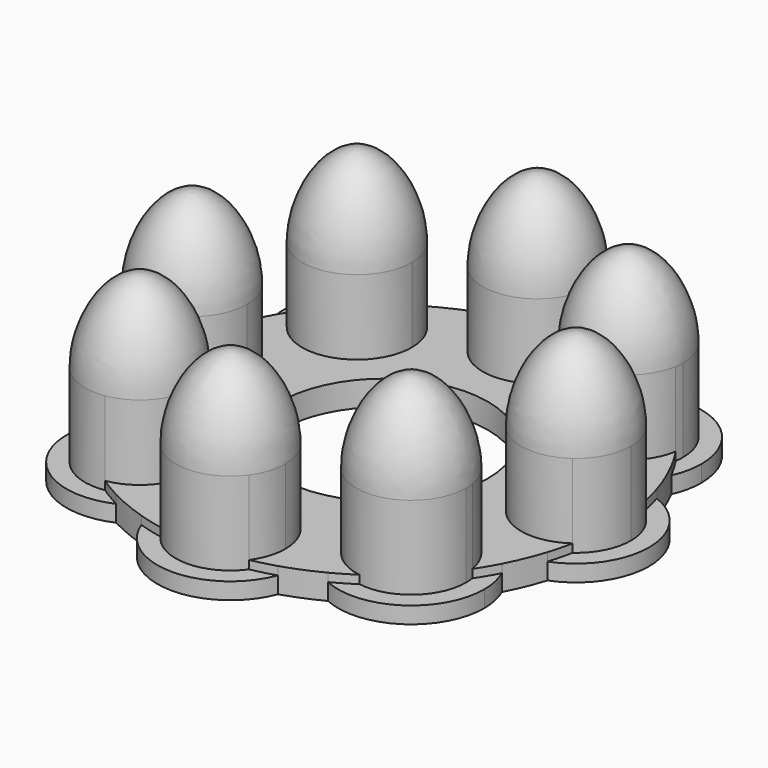
from build123d import *

# Parameters (mm, degrees)
F0_R            = 7.9375
F1_DEPTH        = 0.635
F2_DEPTH        = 1.27
F3_DEPTH        = 6.35
F5_COPIES_COUNT = 8


# Not quite as in the source:
# - a pattern or mirror of a feature is missing from the dataset's text; its kind, count and spacing are read off the source's solid


with BuildPart() as f1:
    # F0 (on Top) → F1 (new body)
    with BuildSketch(Plane.XY):
        with BuildLine():
            ThreePointArc((-5.219470135, 16.6642142857), (-1.0147277679, 9.1734047727), (5.588, 14.6685))
            ThreePointArc((5.588, 14.6685), (5.4950952273, 15.6832277679), (5.219470135, 16.6642142857))
            ThreePointArc((5.219470135, 16.6642142857), (4.3120566918, 16.9217337568), (3.3920620288, 17.1298809524))
            ThreePointArc((3.3920620288, 17.1298809524), (3.986264728, 15.96239896), (4.191, 14.6685))
            ThreePointArc((4.191, 14.6685), (-1.29389896, 10.682235272), (-3.3920620288, 17.1298809524))
            ThreePointArc((-3.3920620288, 17.1298809524), (-4.3120566918, 16.9217337568), (-5.219470135, 16.6642142857))
        make_face()
        with BuildLine():
            ThreePointArc((9.7141049196, 14.5112050451), (8.9163881613, 15.0145572165), (8.0926561979, 15.4741016512))
            ThreePointArc((8.0926561979, 15.4741016512), (6.4208831266, 6.4208831266), (15.4741016512, 8.0926561979))
            ThreePointArc((15.4741016512, 8.0926561979), (15.0145572165, 8.9163881613), (14.5112050451, 9.7141049196))
            ThreePointArc((14.5112050451, 9.7141049196), (7.4087112999, 7.4087112999), (9.7141049196, 14.5112050451))
        make_face()
        with BuildLine():
            ThreePointArc((17.1298809524, 3.3920620288), (16.9217337568, 4.3120566918), (16.6642142857, 5.219470135))
            ThreePointArc((16.6642142857, 5.219470135), (9.0805, 0), (16.6642142857, -5.219470135))
            ThreePointArc((16.6642142857, -5.219470135), (16.9217337568, -4.3120566918), (17.1298809524, -3.3920620288))
            ThreePointArc((17.1298809524, -3.3920620288), (10.4775, 0), (17.1298809524, 3.3920620288))
        make_face()
        with BuildLine():
            ThreePointArc((14.5112050451, -9.7141049196), (15.0145572165, -8.9163881613), (15.4741016512, -8.0926561979))
            ThreePointArc((15.4741016512, -8.0926561979), (6.4208831266, -6.4208831266), (8.0926561979, -15.4741016512))
            ThreePointArc((8.0926561979, -15.4741016512), (8.9163881613, -15.0145572165), (9.7141049196, -14.5112050451))
            ThreePointArc((9.7141049196, -14.5112050451), (7.4087112999, -7.4087112999), (14.5112050451, -9.7141049196))
        make_face()
        with BuildLine():
            ThreePointArc((3.3920620288, -17.1298809524), (4.3120566918, -16.9217337568), (5.219470135, -16.6642142857))
            ThreePointArc((5.219470135, -16.6642142857), (5.4950952273, -15.6832277679), (5.588, -14.6685))
            ThreePointArc((5.588, -14.6685), (-1.0147277679, -9.1734047727), (-5.219470135, -16.6642142857))
            ThreePointArc((-5.219470135, -16.6642142857), (-4.3120566918, -16.9217337568), (-3.3920620288, -17.1298809524))
            ThreePointArc((-3.3920620288, -17.1298809524), (-1.29389896, -10.682235272), (4.191, -14.6685))
            ThreePointArc((4.191, -14.6685), (3.986264728, -15.96239896), (3.3920620288, -17.1298809524))
        make_face()
        with BuildLine():
            ThreePointArc((-4.7841958198, -10.3721958198), (-9.2068001329, -4.907070305), (-15.4741016512, -8.0926561979))
            ThreePointArc((-15.4741016512, -8.0926561979), (-15.0145572165, -8.9163881613), (-14.5112050451, -9.7141049196))
            ThreePointArc((-14.5112050451, -9.7141049196), (-10.0421251177, -6.1942137314), (-6.1811958198, -10.3721958198))
            ThreePointArc((-6.1811958198, -10.3721958198), (-7.1845211216, -13.0930800545), (-9.7141049196, -14.5112050451))
            ThreePointArc((-9.7141049196, -14.5112050451), (-8.9163881613, -15.0145572165), (-8.0926561979, -15.4741016512))
            ThreePointArc((-8.0926561979, -15.4741016512), (-5.6837093153, -13.4125639384), (-4.7841958198, -10.3721958198))
        make_face()
        with BuildLine():
            ThreePointArc((-9.0805, 0), (-11.5004017872, 4.6031399842), (-16.6642142857, 5.219470135))
            ThreePointArc((-16.6642142857, 5.219470135), (-16.9217337568, 4.3120566918), (-17.1298809524, 3.3920620288))
            ThreePointArc((-17.1298809524, 3.3920620288), (-12.764709908, 3.7336395495), (-10.4775, 0))
            ThreePointArc((-10.4775, 0), (-12.764709908, -3.7336395495), (-17.1298809524, -3.3920620288))
            ThreePointArc((-17.1298809524, -3.3920620288), (-16.9217337568, -4.3120566918), (-16.6642142857, -5.219470135))
            ThreePointArc((-16.6642142857, -5.219470135), (-11.5004017872, -4.6031399842), (-9.0805, 0))
        make_face()
        with BuildLine():
            ThreePointArc((-4.7841958198, 10.3721958198), (-5.6837093153, 13.4125639384), (-8.0926561979, 15.4741016512))
            ThreePointArc((-8.0926561979, 15.4741016512), (-8.9163881613, 15.0145572165), (-9.7141049196, 14.5112050451))
            ThreePointArc((-9.7141049196, 14.5112050451), (-7.1845211216, 13.0930800545), (-6.1811958198, 10.3721958198))
            ThreePointArc((-6.1811958198, 10.3721958198), (-10.0421251177, 6.1942137314), (-14.5112050451, 9.7141049196))
            ThreePointArc((-14.5112050451, 9.7141049196), (-15.0145572165, 8.9163881613), (-15.4741016512, 8.0926561979))
            ThreePointArc((-15.4741016512, 8.0926561979), (-9.2068001329, 4.907070305), (-4.7841958198, 10.3721958198))
        make_face()
        with BuildLine():
            ThreePointArc((5.219470135, 16.6642142857), (5.4950952273, 15.6832277679), (5.588, 14.6685))
            ThreePointArc((5.588, 14.6685), (-1.0147277679, 9.1734047727), (-5.219470135, 16.6642142857))
            ThreePointArc((-5.219470135, 16.6642142857), (-6.6826094377, 16.1332463365), (-8.0926561979, 15.4741016512))
            ThreePointArc((-8.0926561979, 15.4741016512), (-5.6837093153, 13.4125639384), (-4.7841958198, 10.3721958198))
            ThreePointArc((-4.7841958198, 10.3721958198), (-9.2068001329, 4.907070305), (-15.4741016512, 8.0926561979))
            ThreePointArc((-15.4741016512, 8.0926561979), (-16.1332463365, 6.6826094377), (-16.6642142857, 5.219470135))
            ThreePointArc((-16.6642142857, 5.219470135), (-11.5004017872, 4.6031399842), (-9.0805, 0))
            ThreePointArc((-9.0805, 0), (-11.5004017872, -4.6031399842), (-16.6642142857, -5.219470135))
            ThreePointArc((-16.6642142857, -5.219470135), (-16.1332463365, -6.6826094377), (-15.4741016512, -8.0926561979))
            ThreePointArc((-15.4741016512, -8.0926561979), (-9.2068001329, -4.907070305), (-4.7841958198, -10.3721958198))
            ThreePointArc((-4.7841958198, -10.3721958198), (-5.6837093153, -13.4125639384), (-8.0926561979, -15.4741016512))
            ThreePointArc((-8.0926561979, -15.4741016512), (-6.6826094377, -16.1332463365), (-5.219470135, -16.6642142857))
            ThreePointArc((-5.219470135, -16.6642142857), (-1.0147277679, -9.1734047727), (5.588, -14.6685))
            ThreePointArc((5.588, -14.6685), (5.4950952273, -15.6832277679), (5.219470135, -16.6642142857))
            ThreePointArc((5.219470135, -16.6642142857), (6.6826094377, -16.1332463365), (8.0926561979, -15.4741016512))
            ThreePointArc((8.0926561979, -15.4741016512), (6.4208831266, -6.4208831266), (15.4741016512, -8.0926561979))
            ThreePointArc((15.4741016512, -8.0926561979), (16.1332463365, -6.6826094377), (16.6642142857, -5.219470135))
            ThreePointArc((16.6642142857, -5.219470135), (9.0805, 0), (16.6642142857, 5.219470135))
            ThreePointArc((16.6642142857, 5.219470135), (16.1332463365, 6.6826094377), (15.4741016512, 8.0926561979))
            ThreePointArc((15.4741016512, 8.0926561979), (6.4208831266, 6.4208831266), (8.0926561979, 15.4741016512))
            ThreePointArc((8.0926561979, 15.4741016512), (6.6826094377, 16.1332463365), (5.219470135, 16.6642142857))
        make_face()
        Circle(F0_R, mode=Mode.SUBTRACT)
    extrude(amount=F1_DEPTH)

    # F0 (on Top) → F2 (join)
    with BuildSketch(Plane.XY):
        with BuildLine():
            ThreePointArc((-5.219470135, 16.6642142857), (-1.0147277679, 9.1734047727), (5.588, 14.6685))
            ThreePointArc((5.588, 14.6685), (5.4950952273, 15.6832277679), (5.219470135, 16.6642142857))
            ThreePointArc((5.219470135, 16.6642142857), (4.3120566918, 16.9217337568), (3.3920620288, 17.1298809524))
            ThreePointArc((3.3920620288, 17.1298809524), (3.986264728, 15.96239896), (4.191, 14.6685))
            ThreePointArc((4.191, 14.6685), (-1.29389896, 10.682235272), (-3.3920620288, 17.1298809524))
            ThreePointArc((-3.3920620288, 17.1298809524), (-4.3120566918, 16.9217337568), (-5.219470135, 16.6642142857))
        make_face()
        with BuildLine():
            ThreePointArc((5.219470135, 16.6642142857), (5.4950952273, 15.6832277679), (5.588, 14.6685))
            ThreePointArc((5.588, 14.6685), (-1.0147277679, 9.1734047727), (-5.219470135, 16.6642142857))
            ThreePointArc((-5.219470135, 16.6642142857), (-6.6826094377, 16.1332463365), (-8.0926561979, 15.4741016512))
            ThreePointArc((-8.0926561979, 15.4741016512), (-5.6837093153, 13.4125639384), (-4.7841958198, 10.3721958198))
            ThreePointArc((-4.7841958198, 10.3721958198), (-9.2068001329, 4.907070305), (-15.4741016512, 8.0926561979))
            ThreePointArc((-15.4741016512, 8.0926561979), (-16.1332463365, 6.6826094377), (-16.6642142857, 5.219470135))
            ThreePointArc((-16.6642142857, 5.219470135), (-11.5004017872, 4.6031399842), (-9.0805, 0))
            ThreePointArc((-9.0805, 0), (-11.5004017872, -4.6031399842), (-16.6642142857, -5.219470135))
            ThreePointArc((-16.6642142857, -5.219470135), (-16.1332463365, -6.6826094377), (-15.4741016512, -8.0926561979))
            ThreePointArc((-15.4741016512, -8.0926561979), (-9.2068001329, -4.907070305), (-4.7841958198, -10.3721958198))
            ThreePointArc((-4.7841958198, -10.3721958198), (-5.6837093153, -13.4125639384), (-8.0926561979, -15.4741016512))
            ThreePointArc((-8.0926561979, -15.4741016512), (-6.6826094377, -16.1332463365), (-5.219470135, -16.6642142857))
            ThreePointArc((-5.219470135, -16.6642142857), (-1.0147277679, -9.1734047727), (5.588, -14.6685))
            ThreePointArc((5.588, -14.6685), (5.4950952273, -15.6832277679), (5.219470135, -16.6642142857))
            ThreePointArc((5.219470135, -16.6642142857), (6.6826094377, -16.1332463365), (8.0926561979, -15.4741016512))
            ThreePointArc((8.0926561979, -15.4741016512), (6.4208831266, -6.4208831266), (15.4741016512, -8.0926561979))
            ThreePointArc((15.4741016512, -8.0926561979), (16.1332463365, -6.6826094377), (16.6642142857, -5.219470135))
            ThreePointArc((16.6642142857, -5.219470135), (9.0805, 0), (16.6642142857, 5.219470135))
            ThreePointArc((16.6642142857, 5.219470135), (16.1332463365, 6.6826094377), (15.4741016512, 8.0926561979))
            ThreePointArc((15.4741016512, 8.0926561979), (6.4208831266, 6.4208831266), (8.0926561979, 15.4741016512))
            ThreePointArc((8.0926561979, 15.4741016512), (6.6826094377, 16.1332463365), (5.219470135, 16.6642142857))
        make_face()
        Circle(F0_R, mode=Mode.SUBTRACT)
        with BuildLine():
            ThreePointArc((3.3920620288, 17.1298809524), (4.3120566918, 16.9217337568), (5.219470135, 16.6642142857))
            ThreePointArc((5.219470135, 16.6642142857), (0, 20.2565), (-5.219470135, 16.6642142857))
            ThreePointArc((-5.219470135, 16.6642142857), (-4.3120566918, 16.9217337568), (-3.3920620288, 17.1298809524))
            ThreePointArc((-3.3920620288, 17.1298809524), (0, 18.8595), (3.3920620288, 17.1298809524))
        make_face()
        with BuildLine():
            ThreePointArc((15.9601958198, 10.3721958198), (13.4125639384, 15.0606823244), (8.0926561979, 15.4741016512))
            ThreePointArc((8.0926561979, 15.4741016512), (8.9163881613, 15.0145572165), (9.7141049196, 14.5112050451))
            ThreePointArc((9.7141049196, 14.5112050451), (13.0930800545, 13.559870518), (14.5631958198, 10.3721958198))
            ThreePointArc((14.5631958198, 10.3721958198), (14.5501779083, 10.0421251177), (14.5112050451, 9.7141049196))
            ThreePointArc((14.5112050451, 9.7141049196), (15.0145572165, 8.9163881613), (15.4741016512, 8.0926561979))
            ThreePointArc((15.4741016512, 8.0926561979), (15.8373213347, 9.2068001329), (15.9601958198, 10.3721958198))
        make_face()
        with BuildLine():
            ThreePointArc((9.7141049196, 14.5112050451), (8.9163881613, 15.0145572165), (8.0926561979, 15.4741016512))
            ThreePointArc((8.0926561979, 15.4741016512), (6.4208831266, 6.4208831266), (15.4741016512, 8.0926561979))
            ThreePointArc((15.4741016512, 8.0926561979), (15.0145572165, 8.9163881613), (14.5112050451, 9.7141049196))
            ThreePointArc((14.5112050451, 9.7141049196), (7.4087112999, 7.4087112999), (9.7141049196, 14.5112050451))
        make_face()
        with BuildLine():
            ThreePointArc((-4.7841958198, 10.3721958198), (-5.6837093153, 13.4125639384), (-8.0926561979, 15.4741016512))
            ThreePointArc((-8.0926561979, 15.4741016512), (-8.9163881613, 15.0145572165), (-9.7141049196, 14.5112050451))
            ThreePointArc((-9.7141049196, 14.5112050451), (-7.1845211216, 13.0930800545), (-6.1811958198, 10.3721958198))
            ThreePointArc((-6.1811958198, 10.3721958198), (-10.0421251177, 6.1942137314), (-14.5112050451, 9.7141049196))
            ThreePointArc((-14.5112050451, 9.7141049196), (-15.0145572165, 8.9163881613), (-15.4741016512, 8.0926561979))
            ThreePointArc((-15.4741016512, 8.0926561979), (-9.2068001329, 4.907070305), (-4.7841958198, 10.3721958198))
        make_face()
        with BuildLine():
            ThreePointArc((-9.7141049196, 14.5112050451), (-8.9163881613, 15.0145572165), (-8.0926561979, 15.4741016512))
            ThreePointArc((-8.0926561979, 15.4741016512), (-14.3235085131, 14.3235085131), (-15.4741016512, 8.0926561979))
            ThreePointArc((-15.4741016512, 8.0926561979), (-15.0145572165, 8.9163881613), (-14.5112050451, 9.7141049196))
            ThreePointArc((-14.5112050451, 9.7141049196), (-13.3356803398, 13.3356803398), (-9.7141049196, 14.5112050451))
        make_face()
        with BuildLine():
            ThreePointArc((20.2565, 0), (19.2716399842, 3.1680982128), (16.6642142857, 5.219470135))
            ThreePointArc((16.6642142857, 5.219470135), (16.9217337568, 4.3120566918), (17.1298809524, 3.3920620288))
            ThreePointArc((17.1298809524, 3.3920620288), (18.4021395495, 1.903790092), (18.8595, 0))
            ThreePointArc((18.8595, 0), (18.4021395495, -1.903790092), (17.1298809524, -3.3920620288))
            ThreePointArc((17.1298809524, -3.3920620288), (16.9217337568, -4.3120566918), (16.6642142857, -5.219470135))
            ThreePointArc((16.6642142857, -5.219470135), (19.2716399842, -3.1680982128), (20.2565, 0))
        make_face()
        with BuildLine():
            ThreePointArc((17.1298809524, 3.3920620288), (16.9217337568, 4.3120566918), (16.6642142857, 5.219470135))
            ThreePointArc((16.6642142857, 5.219470135), (9.0805, 0), (16.6642142857, -5.219470135))
            ThreePointArc((16.6642142857, -5.219470135), (16.9217337568, -4.3120566918), (17.1298809524, -3.3920620288))
            ThreePointArc((17.1298809524, -3.3920620288), (10.4775, 0), (17.1298809524, 3.3920620288))
        make_face()
        with BuildLine():
            ThreePointArc((-9.0805, 0), (-11.5004017872, 4.6031399842), (-16.6642142857, 5.219470135))
            ThreePointArc((-16.6642142857, 5.219470135), (-16.9217337568, 4.3120566918), (-17.1298809524, 3.3920620288))
            ThreePointArc((-17.1298809524, 3.3920620288), (-12.764709908, 3.7336395495), (-10.4775, 0))
            ThreePointArc((-10.4775, 0), (-12.764709908, -3.7336395495), (-17.1298809524, -3.3920620288))
            ThreePointArc((-17.1298809524, -3.3920620288), (-16.9217337568, -4.3120566918), (-16.6642142857, -5.219470135))
            ThreePointArc((-16.6642142857, -5.219470135), (-11.5004017872, -4.6031399842), (-9.0805, 0))
        make_face()
        with BuildLine():
            ThreePointArc((-17.1298809524, 3.3920620288), (-16.9217337568, 4.3120566918), (-16.6642142857, 5.219470135))
            ThreePointArc((-16.6642142857, 5.219470135), (-20.2565, 0), (-16.6642142857, -5.219470135))
            ThreePointArc((-16.6642142857, -5.219470135), (-16.9217337568, -4.3120566918), (-17.1298809524, -3.3920620288))
            ThreePointArc((-17.1298809524, -3.3920620288), (-18.8595, 0), (-17.1298809524, 3.3920620288))
        make_face()
        with BuildLine():
            ThreePointArc((15.9601958198, -10.3721958198), (15.8373213347, -9.2068001329), (15.4741016512, -8.0926561979))
            ThreePointArc((15.4741016512, -8.0926561979), (15.0145572165, -8.9163881613), (14.5112050451, -9.7141049196))
            ThreePointArc((14.5112050451, -9.7141049196), (14.5501779083, -10.0421251177), (14.5631958198, -10.3721958198))
            ThreePointArc((14.5631958198, -10.3721958198), (13.0930800545, -13.559870518), (9.7141049196, -14.5112050451))
            ThreePointArc((9.7141049196, -14.5112050451), (8.9163881613, -15.0145572165), (8.0926561979, -15.4741016512))
            ThreePointArc((8.0926561979, -15.4741016512), (13.4125639384, -15.0606823244), (15.9601958198, -10.3721958198))
        make_face()
        with BuildLine():
            ThreePointArc((14.5112050451, -9.7141049196), (15.0145572165, -8.9163881613), (15.4741016512, -8.0926561979))
            ThreePointArc((15.4741016512, -8.0926561979), (6.4208831266, -6.4208831266), (8.0926561979, -15.4741016512))
            ThreePointArc((8.0926561979, -15.4741016512), (8.9163881613, -15.0145572165), (9.7141049196, -14.5112050451))
            ThreePointArc((9.7141049196, -14.5112050451), (7.4087112999, -7.4087112999), (14.5112050451, -9.7141049196))
        make_face()
        with BuildLine():
            ThreePointArc((-4.7841958198, -10.3721958198), (-9.2068001329, -4.907070305), (-15.4741016512, -8.0926561979))
            ThreePointArc((-15.4741016512, -8.0926561979), (-15.0145572165, -8.9163881613), (-14.5112050451, -9.7141049196))
            ThreePointArc((-14.5112050451, -9.7141049196), (-10.0421251177, -6.1942137314), (-6.1811958198, -10.3721958198))
            ThreePointArc((-6.1811958198, -10.3721958198), (-7.1845211216, -13.0930800545), (-9.7141049196, -14.5112050451))
            ThreePointArc((-9.7141049196, -14.5112050451), (-8.9163881613, -15.0145572165), (-8.0926561979, -15.4741016512))
            ThreePointArc((-8.0926561979, -15.4741016512), (-5.6837093153, -13.4125639384), (-4.7841958198, -10.3721958198))
        make_face()
        with BuildLine():
            ThreePointArc((-14.5112050451, -9.7141049196), (-15.0145572165, -8.9163881613), (-15.4741016512, -8.0926561979))
            ThreePointArc((-15.4741016512, -8.0926561979), (-14.3235085131, -14.3235085131), (-8.0926561979, -15.4741016512))
            ThreePointArc((-8.0926561979, -15.4741016512), (-8.9163881613, -15.0145572165), (-9.7141049196, -14.5112050451))
            ThreePointArc((-9.7141049196, -14.5112050451), (-13.3356803398, -13.3356803398), (-14.5112050451, -9.7141049196))
        make_face()
        with BuildLine():
            ThreePointArc((-5.219470135, -16.6642142857), (0, -20.2565), (5.219470135, -16.6642142857))
            ThreePointArc((5.219470135, -16.6642142857), (4.3120566918, -16.9217337568), (3.3920620288, -17.1298809524))
            ThreePointArc((3.3920620288, -17.1298809524), (0, -18.8595), (-3.3920620288, -17.1298809524))
            ThreePointArc((-3.3920620288, -17.1298809524), (-4.3120566918, -16.9217337568), (-5.219470135, -16.6642142857))
        make_face()
        with BuildLine():
            ThreePointArc((3.3920620288, -17.1298809524), (4.3120566918, -16.9217337568), (5.219470135, -16.6642142857))
            ThreePointArc((5.219470135, -16.6642142857), (5.4950952273, -15.6832277679), (5.588, -14.6685))
            ThreePointArc((5.588, -14.6685), (-1.0147277679, -9.1734047727), (-5.219470135, -16.6642142857))
            ThreePointArc((-5.219470135, -16.6642142857), (-4.3120566918, -16.9217337568), (-3.3920620288, -17.1298809524))
            ThreePointArc((-3.3920620288, -17.1298809524), (-1.29389896, -10.682235272), (4.191, -14.6685))
            ThreePointArc((4.191, -14.6685), (3.986264728, -15.96239896), (3.3920620288, -17.1298809524))
        make_face()
        with BuildLine():
            ThreePointArc((-3.3920620288, -17.1298809524), (0, -18.8595), (3.3920620288, -17.1298809524))
            ThreePointArc((3.3920620288, -17.1298809524), (0, -17.4625), (-3.3920620288, -17.1298809524))
        make_face()
        with BuildLine():
            ThreePointArc((-3.3920620288, -17.1298809524), (0, -17.4625), (3.3920620288, -17.1298809524))
            ThreePointArc((3.3920620288, -17.1298809524), (3.986264728, -15.96239896), (4.191, -14.6685))
            ThreePointArc((4.191, -14.6685), (-1.29389896, -10.682235272), (-3.3920620288, -17.1298809524))
        make_face()
        with BuildLine():
            ThreePointArc((9.7141049196, -14.5112050451), (12.3478521665, -12.3478521665), (14.5112050451, -9.7141049196))
            ThreePointArc((14.5112050451, -9.7141049196), (7.4087112999, -7.4087112999), (9.7141049196, -14.5112050451))
        make_face()
        with BuildLine():
            ThreePointArc((14.5631958198, -10.3721958198), (14.5501779083, -10.0421251177), (14.5112050451, -9.7141049196))
            ThreePointArc((14.5112050451, -9.7141049196), (12.3478521665, -12.3478521665), (9.7141049196, -14.5112050451))
            ThreePointArc((9.7141049196, -14.5112050451), (13.0930800545, -13.559870518), (14.5631958198, -10.3721958198))
        make_face()
        with BuildLine():
            ThreePointArc((18.8595, 0), (18.4021395495, 1.903790092), (17.1298809524, 3.3920620288))
            ThreePointArc((17.1298809524, 3.3920620288), (17.3791463021, 1.7041655024), (17.4625, 0))
            ThreePointArc((17.4625, 0), (17.3791463021, -1.7041655024), (17.1298809524, -3.3920620288))
            ThreePointArc((17.1298809524, -3.3920620288), (18.4021395495, -1.903790092), (18.8595, 0))
        make_face()
        with BuildLine():
            ThreePointArc((17.4625, 0), (17.3791463021, 1.7041655024), (17.1298809524, 3.3920620288))
            ThreePointArc((17.1298809524, 3.3920620288), (10.4775, 0), (17.1298809524, -3.3920620288))
            ThreePointArc((17.1298809524, -3.3920620288), (17.3791463021, -1.7041655024), (17.4625, 0))
        make_face()
        with BuildLine():
            ThreePointArc((14.5112050451, 9.7141049196), (12.3478521665, 12.3478521665), (9.7141049196, 14.5112050451))
            ThreePointArc((9.7141049196, 14.5112050451), (7.4087112999, 7.4087112999), (14.5112050451, 9.7141049196))
        make_face()
        with BuildLine():
            ThreePointArc((14.5631958198, 10.3721958198), (13.0930800545, 13.559870518), (9.7141049196, 14.5112050451))
            ThreePointArc((9.7141049196, 14.5112050451), (12.3478521665, 12.3478521665), (14.5112050451, 9.7141049196))
            ThreePointArc((14.5112050451, 9.7141049196), (14.5501779083, 10.0421251177), (14.5631958198, 10.3721958198))
        make_face()
        with BuildLine():
            ThreePointArc((-6.1811958198, 10.3721958198), (-7.1845211216, 13.0930800545), (-9.7141049196, 14.5112050451))
            ThreePointArc((-9.7141049196, 14.5112050451), (-12.3478521665, 12.3478521665), (-14.5112050451, 9.7141049196))
            ThreePointArc((-14.5112050451, 9.7141049196), (-10.0421251177, 6.1942137314), (-6.1811958198, 10.3721958198))
        make_face()
        with BuildLine():
            ThreePointArc((-14.5112050451, 9.7141049196), (-12.3478521665, 12.3478521665), (-9.7141049196, 14.5112050451))
            ThreePointArc((-9.7141049196, 14.5112050451), (-13.3356803398, 13.3356803398), (-14.5112050451, 9.7141049196))
        make_face()
        with BuildLine():
            ThreePointArc((-10.4775, 0), (-12.764709908, 3.7336395495), (-17.1298809524, 3.3920620288))
            ThreePointArc((-17.1298809524, 3.3920620288), (-17.4625, 0), (-17.1298809524, -3.3920620288))
            ThreePointArc((-17.1298809524, -3.3920620288), (-12.764709908, -3.7336395495), (-10.4775, 0))
        make_face()
        with BuildLine():
            ThreePointArc((4.191, 14.6685), (3.986264728, 15.96239896), (3.3920620288, 17.1298809524))
            ThreePointArc((3.3920620288, 17.1298809524), (0, 17.4625), (-3.3920620288, 17.1298809524))
            ThreePointArc((-3.3920620288, 17.1298809524), (-1.29389896, 10.682235272), (4.191, 14.6685))
        make_face()
        with BuildLine():
            ThreePointArc((-3.3920620288, 17.1298809524), (0, 17.4625), (3.3920620288, 17.1298809524))
            ThreePointArc((3.3920620288, 17.1298809524), (0, 18.8595), (-3.3920620288, 17.1298809524))
        make_face()
        with BuildLine():
            ThreePointArc((-9.7141049196, -14.5112050451), (-12.3478521665, -12.3478521665), (-14.5112050451, -9.7141049196))
            ThreePointArc((-14.5112050451, -9.7141049196), (-13.3356803398, -13.3356803398), (-9.7141049196, -14.5112050451))
        make_face()
        with BuildLine():
            ThreePointArc((-6.1811958198, -10.3721958198), (-10.0421251177, -6.1942137314), (-14.5112050451, -9.7141049196))
            ThreePointArc((-14.5112050451, -9.7141049196), (-12.3478521665, -12.3478521665), (-9.7141049196, -14.5112050451))
            ThreePointArc((-9.7141049196, -14.5112050451), (-7.1845211216, -13.0930800545), (-6.1811958198, -10.3721958198))
        make_face()
        with BuildLine():
            ThreePointArc((-17.1298809524, -3.3920620288), (-17.4625, 0), (-17.1298809524, 3.3920620288))
            ThreePointArc((-17.1298809524, 3.3920620288), (-18.8595, 0), (-17.1298809524, -3.3920620288))
        make_face()
    extrude(amount=-F2_DEPTH)

    # F0 (on Top) → F3 (join)
    with BuildSketch(Plane.XY):
        with BuildLine():
            ThreePointArc((9.7141049196, -14.5112050451), (12.3478521665, -12.3478521665), (14.5112050451, -9.7141049196))
            ThreePointArc((14.5112050451, -9.7141049196), (7.4087112999, -7.4087112999), (9.7141049196, -14.5112050451))
        make_face()
        with BuildLine():
            ThreePointArc((14.5631958198, -10.3721958198), (14.5501779083, -10.0421251177), (14.5112050451, -9.7141049196))
            ThreePointArc((14.5112050451, -9.7141049196), (12.3478521665, -12.3478521665), (9.7141049196, -14.5112050451))
            ThreePointArc((9.7141049196, -14.5112050451), (13.0930800545, -13.559870518), (14.5631958198, -10.3721958198))
        make_face()
        with BuildLine():
            ThreePointArc((-3.3920620288, -17.1298809524), (0, -18.8595), (3.3920620288, -17.1298809524))
            ThreePointArc((3.3920620288, -17.1298809524), (0, -17.4625), (-3.3920620288, -17.1298809524))
        make_face()
        with BuildLine():
            ThreePointArc((-3.3920620288, -17.1298809524), (0, -17.4625), (3.3920620288, -17.1298809524))
            ThreePointArc((3.3920620288, -17.1298809524), (3.986264728, -15.96239896), (4.191, -14.6685))
            ThreePointArc((4.191, -14.6685), (-1.29389896, -10.682235272), (-3.3920620288, -17.1298809524))
        make_face()
        with BuildLine():
            ThreePointArc((-6.1811958198, -10.3721958198), (-10.0421251177, -6.1942137314), (-14.5112050451, -9.7141049196))
            ThreePointArc((-14.5112050451, -9.7141049196), (-12.3478521665, -12.3478521665), (-9.7141049196, -14.5112050451))
            ThreePointArc((-9.7141049196, -14.5112050451), (-7.1845211216, -13.0930800545), (-6.1811958198, -10.3721958198))
        make_face()
        with BuildLine():
            ThreePointArc((-9.7141049196, -14.5112050451), (-12.3478521665, -12.3478521665), (-14.5112050451, -9.7141049196))
            ThreePointArc((-14.5112050451, -9.7141049196), (-13.3356803398, -13.3356803398), (-9.7141049196, -14.5112050451))
        make_face()
        with BuildLine():
            ThreePointArc((-10.4775, 0), (-12.764709908, 3.7336395495), (-17.1298809524, 3.3920620288))
            ThreePointArc((-17.1298809524, 3.3920620288), (-17.4625, 0), (-17.1298809524, -3.3920620288))
            ThreePointArc((-17.1298809524, -3.3920620288), (-12.764709908, -3.7336395495), (-10.4775, 0))
        make_face()
        with BuildLine():
            ThreePointArc((-17.1298809524, -3.3920620288), (-17.4625, 0), (-17.1298809524, 3.3920620288))
            ThreePointArc((-17.1298809524, 3.3920620288), (-18.8595, 0), (-17.1298809524, -3.3920620288))
        make_face()
        with BuildLine():
            ThreePointArc((-6.1811958198, 10.3721958198), (-7.1845211216, 13.0930800545), (-9.7141049196, 14.5112050451))
            ThreePointArc((-9.7141049196, 14.5112050451), (-12.3478521665, 12.3478521665), (-14.5112050451, 9.7141049196))
            ThreePointArc((-14.5112050451, 9.7141049196), (-10.0421251177, 6.1942137314), (-6.1811958198, 10.3721958198))
        make_face()
        with BuildLine():
            ThreePointArc((-14.5112050451, 9.7141049196), (-12.3478521665, 12.3478521665), (-9.7141049196, 14.5112050451))
            ThreePointArc((-9.7141049196, 14.5112050451), (-13.3356803398, 13.3356803398), (-14.5112050451, 9.7141049196))
        make_face()
        with BuildLine():
            ThreePointArc((4.191, 14.6685), (3.986264728, 15.96239896), (3.3920620288, 17.1298809524))
            ThreePointArc((3.3920620288, 17.1298809524), (0, 17.4625), (-3.3920620288, 17.1298809524))
            ThreePointArc((-3.3920620288, 17.1298809524), (-1.29389896, 10.682235272), (4.191, 14.6685))
        make_face()
        with BuildLine():
            ThreePointArc((-3.3920620288, 17.1298809524), (0, 17.4625), (3.3920620288, 17.1298809524))
            ThreePointArc((3.3920620288, 17.1298809524), (0, 18.8595), (-3.3920620288, 17.1298809524))
        make_face()
        with BuildLine():
            ThreePointArc((14.5112050451, 9.7141049196), (12.3478521665, 12.3478521665), (9.7141049196, 14.5112050451))
            ThreePointArc((9.7141049196, 14.5112050451), (7.4087112999, 7.4087112999), (14.5112050451, 9.7141049196))
        make_face()
        with BuildLine():
            ThreePointArc((14.5631958198, 10.3721958198), (13.0930800545, 13.559870518), (9.7141049196, 14.5112050451))
            ThreePointArc((9.7141049196, 14.5112050451), (12.3478521665, 12.3478521665), (14.5112050451, 9.7141049196))
            ThreePointArc((14.5112050451, 9.7141049196), (14.5501779083, 10.0421251177), (14.5631958198, 10.3721958198))
        make_face()
        with BuildLine():
            ThreePointArc((17.4625, 0), (17.3791463021, 1.7041655024), (17.1298809524, 3.3920620288))
            ThreePointArc((17.1298809524, 3.3920620288), (10.4775, 0), (17.1298809524, -3.3920620288))
            ThreePointArc((17.1298809524, -3.3920620288), (17.3791463021, -1.7041655024), (17.4625, 0))
        make_face()
        with BuildLine():
            ThreePointArc((18.8595, 0), (18.4021395495, 1.903790092), (17.1298809524, 3.3920620288))
            ThreePointArc((17.1298809524, 3.3920620288), (17.3791463021, 1.7041655024), (17.4625, 0))
            ThreePointArc((17.4625, 0), (17.3791463021, -1.7041655024), (17.1298809524, -3.3920620288))
            ThreePointArc((17.1298809524, -3.3920620288), (18.4021395495, -1.903790092), (18.8595, 0))
        make_face()
    extrude(amount=F3_DEPTH)

    # F4 (on Right) → F5 (revolve)
    with BuildSketch(Plane.YZ):
        with BuildLine():
            Line((14.6685, 12.7), (14.6685, 6.35))
            Line((14.6685, 6.35), (18.8595, 6.35))
            add(Edge.make_bspline(
                [(14.6685, 12.7), (16.764, 12.7), (18.8595, 9.525), (18.8595, 6.35)],
                knots=[0, 0, 0, 0, 7.6083494268, 7.6083494268, 7.6083494268, 7.6083494268], degree=3))
        make_face()
    f5 = revolve(axis=Axis((0, 14.6685, 9.525), (0, 0, 1)))

    # F5_copies: F5 ×8 about axis
    f5_copies_axis = Axis((0, 0, 0), (0, 0, 1))
    for i in range(1, F5_COPIES_COUNT):
        add(f5.rotate(f5_copies_axis, i * 360 / F5_COPIES_COUNT))


solid = f1.part
